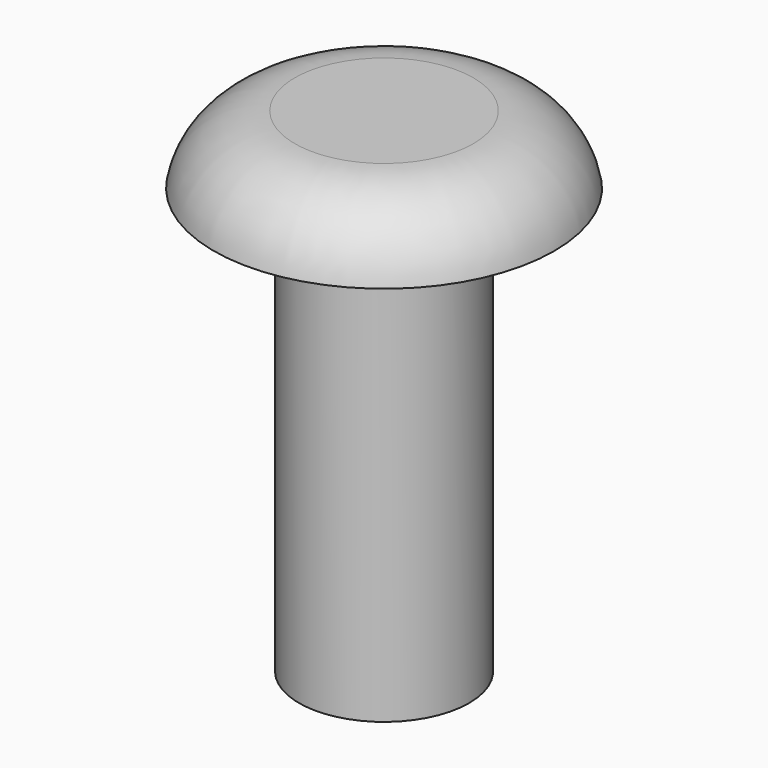
from build123d import *

# Parameters (mm, degrees)
F0_R     = 6.35
F1_DEPTH = 2.54
F3_R     = 3.175
F4_DEPTH = 15.875


# Not quite as in the source:
# - a fillet or chamfer that OpenCascade refuses, or shapes differently, is made with other operations: its cross-section is extruded or revolved along the edge and cut away or added


with BuildPart() as f1:
    # F0 (on Top) → F1 (new body)
    with BuildSketch(Plane.XY):
        Circle(F0_R)
    extrude(amount=F1_DEPTH)

    # F2: fillet of radius 3.0660512242 on 1 edges, made by hand

    # F2_s1 → F2_t2 (revolve, cut)
    with BuildSketch(Plane.XZ):
        with BuildLine():
            ThreePointArc((6.35, 0), (5.3027068749, 1.8206027884), (3.3294139279, 2.54))
            Line((3.3294139279, 2.54), (6.35, 2.54))
            Line((6.35, 2.54), (6.35, 0))
        make_face()
    revolve(axis=Axis((0, 0, 2.54), (0, 0, 1)), mode=Mode.SUBTRACT)

    # F3 (on face) → F4 (join)
    with BuildSketch(Plane(origin=(0, 0, 0), x_dir=(1, 0, 0), z_dir=(0, 0, -1))):
        Circle(F3_R)
    extrude(amount=F4_DEPTH)


solid = f1.part
